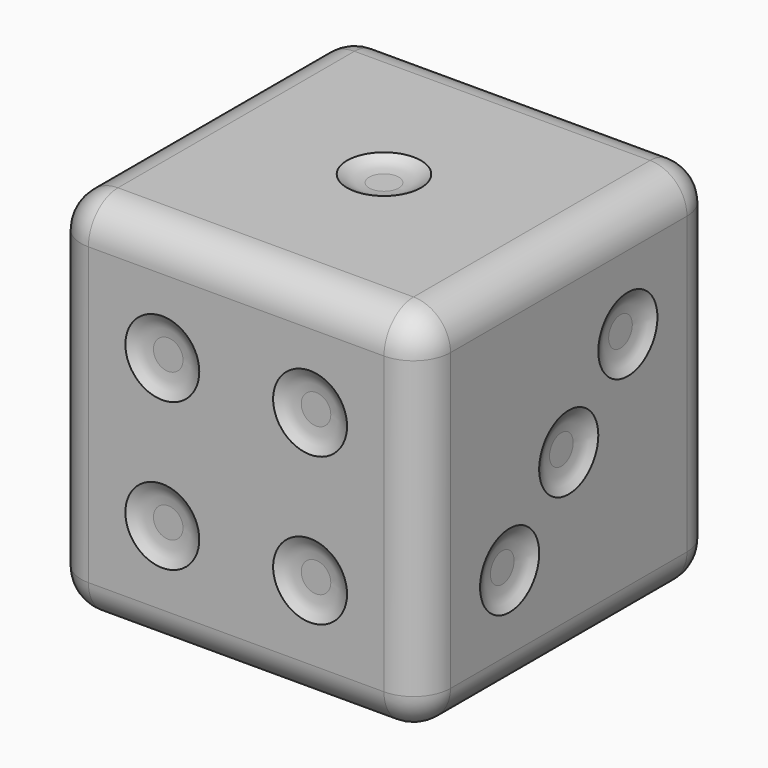
from build123d import *

# Parameters (mm, degrees)
F0_W      = 50
F0_H      = 50
F1_DEPTH  = 50
F2_R      = 5
F3_DEPTH  = 1
F4_R      = 5
F6_R      = 5
F7_DEPTH  = 1
F9_R      = 5
F10_DEPTH = 1
F12_R     = 5
F13_DEPTH = 1
F15_R     = 5
F16_DEPTH = 1
F18_R     = 5
F19_DEPTH = 1
F21_DEPTH = 0.5


# Not quite as in the source:
# - a fillet or chamfer that OpenCascade refuses, or shapes differently, is made with other operations: its cross-section is extruded or revolved along the edge and cut away or added
# - a feature names something its author has since deleted; it is built from what else it names


with BuildPart() as f1:
    # F0 (on Top) → F1 (new body)
    with BuildSketch(Plane.XY):
        with Locations((25, -25)):
            Rectangle(F0_W, F0_H)
    extrude(amount=F1_DEPTH)

    # F2 (on face) → F3 (cut)
    with BuildSketch(Plane.XY.offset(50)):
        with Locations((25, -25)):
            Circle(F2_R)
    extrude(amount=-F3_DEPTH, mode=Mode.SUBTRACT)

    # F4
    f4_edges = [f1.edges().sort_by_distance(p)[0] for p in [
        (0, -50, 25),
        (25, -50, 50),
        (25, 0, 50),
        (0, 0, 25),
        (0, -25, 0),
        (0, -25, 50),
        (25, -50, 0),
        (50, -50, 25),
        (25, 0, 0),
        (50, 0, 25),
        (50, -25, 0),
        (50, -25, 50),
    ]]
    fillet(f4_edges, radius=F4_R)

    # F5: fillet of radius 5 on 1 edges, made by hand

    # F5_s1 → F5_t2 (revolve)
    with BuildSketch(Plane.XZ.offset(25)):
        with BuildLine():
            ThreePointArc((30, 50), (28.5811388301, 49.2565835097), (27, 49))
            Line((27, 49), (30, 49))
            Line((30, 49), (30, 50))
        make_face()
    revolve(axis=Axis((25, -25, 49), (0, 0, 1)))

    # F6 (on face) → F7 (cut)
    with BuildSketch(Plane.XZ.offset(50)):
        with Locations((15, 35)):
            Circle(F6_R)
        with Locations((35, 35)):
            Circle(F6_R)
        with Locations((35, 15)):
            Circle(F6_R)
        with Locations((15, 15)):
            Circle(F6_R)
    extrude(amount=-F7_DEPTH, mode=Mode.SUBTRACT)

    # F8: fillet of radius 5 on 4 edges, made by hand

    # F8_s1 → F8_t2 (revolve)
    with BuildSketch(Plane.XY.offset(35)):
        with BuildLine():
            ThreePointArc((20, -50), (18.5811388301, -49.2565835097), (17, -49))
            Line((17, -49), (20, -49))
            Line((20, -49), (20, -50))
        make_face()
    revolve(axis=Axis((15, -49, 35), (0, -1, 0)))

    # F8_s3 → F8_t4 (revolve)
    with BuildSketch(Plane.XY.offset(35)):
        with BuildLine():
            ThreePointArc((40, -50), (38.5811388301, -49.2565835097), (37, -49))
            Line((37, -49), (40, -49))
            Line((40, -49), (40, -50))
        make_face()
    revolve(axis=Axis((35, -49, 35), (0, -1, 0)))

    # F8_s5 → F8_t6 (revolve)
    with BuildSketch(Plane.XY.offset(15)):
        with BuildLine():
            ThreePointArc((20, -50), (18.5811388301, -49.2565835097), (17, -49))
            Line((17, -49), (20, -49))
            Line((20, -49), (20, -50))
        make_face()
    revolve(axis=Axis((15, -49, 15), (0, -1, 0)))

    # F8_s7 → F8_t8 (revolve)
    with BuildSketch(Plane.XY.offset(15)):
        with BuildLine():
            ThreePointArc((40, -50), (38.5811388301, -49.2565835097), (37, -49))
            Line((37, -49), (40, -49))
            Line((40, -49), (40, -50))
        make_face()
    revolve(axis=Axis((35, -49, 15), (0, -1, 0)))

    # F9 (on face) → F10 (cut)
    with BuildSketch(Plane(origin=(0, 0, 0), x_dir=(-1, 0, 0), z_dir=(0, 1, 0))):
        with Locations((-35, 15)):
            Circle(F9_R)
        with Locations((-15, 35)):
            Circle(F9_R)
    extrude(amount=-F10_DEPTH, mode=Mode.SUBTRACT)

    # F11: fillet of radius 5 on 2 edges, made by hand

    # F11_s1 → F11_t2 (revolve)
    with BuildSketch(Plane.XY.offset(15)):
        with BuildLine():
            ThreePointArc((30, 0), (31.4188611699, -0.7434164903), (33, -1))
            Line((33, -1), (30, -1))
            Line((30, -1), (30, 0))
        make_face()
    revolve(axis=Axis((35, -1, 15), (0, 1, 0)))

    # F11_s3 → F11_t4 (revolve)
    with BuildSketch(Plane.XY.offset(35)):
        with BuildLine():
            ThreePointArc((10, 0), (11.4188611699, -0.7434164903), (13, -1))
            Line((13, -1), (10, -1))
            Line((10, -1), (10, 0))
        make_face()
    revolve(axis=Axis((15, -1, 35), (0, 1, 0)))

    # F12 (on face) → F13 (cut)
    with BuildSketch(Plane.YZ.offset(50)):
        with Locations((-15, 35)):
            Circle(F12_R)
        with Locations((-25, 25)):
            Circle(F12_R)
        with Locations((-35, 15)):
            Circle(F12_R)
    extrude(amount=-F13_DEPTH, mode=Mode.SUBTRACT)

    # F14: fillet of radius 5 on 3 edges, made by hand

    # F14_s1 → F14_t2 (revolve)
    with BuildSketch(Plane.XY.offset(15)):
        with BuildLine():
            ThreePointArc((50, -30), (49.2565835097, -31.4188611699), (49, -33))
            Line((49, -33), (49, -30))
            Line((49, -30), (50, -30))
        make_face()
    revolve(axis=Axis((49, -35, 15), (1, 0, 0)))

    # F14_s3 → F14_t4 (revolve)
    with BuildSketch(Plane.XY.offset(25)):
        with BuildLine():
            ThreePointArc((50, -20), (49.2565835097, -21.4188611699), (49, -23))
            Line((49, -23), (49, -20))
            Line((49, -20), (50, -20))
        make_face()
    revolve(axis=Axis((49, -25, 25), (1, 0, 0)))

    # F14_s5 → F14_t6 (revolve)
    with BuildSketch(Plane.XY.offset(35)):
        with BuildLine():
            ThreePointArc((50, -10), (49.2565835097, -11.4188611699), (49, -13))
            Line((49, -13), (49, -10))
            Line((49, -10), (50, -10))
        make_face()
    revolve(axis=Axis((49, -15, 35), (1, 0, 0)))

    # F15 (on face) → F16 (cut)
    with BuildSketch(Plane(origin=(0, 0, 0), x_dir=(0, -1, 0), z_dir=(-1, 0, 0))):
        with Locations((15, 35)):
            Circle(F15_R)
        with Locations((25, 25)):
            Circle(F15_R)
        with Locations((15, 15)):
            Circle(F15_R)
        with Locations((35, 15)):
            Circle(F15_R)
        with Locations((35, 35)):
            Circle(F15_R)
    extrude(amount=-F16_DEPTH, mode=Mode.SUBTRACT)

    # F17: fillet of radius 5 on 5 edges, made by hand

    # F17_s1 → F17_t2 (revolve)
    with BuildSketch(Plane.XY.offset(35)):
        with BuildLine():
            ThreePointArc((0, -20), (0.7434164903, -18.5811388301), (1, -17))
            Line((1, -17), (1, -20))
            Line((1, -20), (0, -20))
        make_face()
    revolve(axis=Axis((1, -15, 35), (-1, 0, 0)))

    # F17_s3 → F17_t4 (revolve)
    with BuildSketch(Plane.XY.offset(25)):
        with BuildLine():
            ThreePointArc((0, -30), (0.7434164903, -28.5811388301), (1, -27))
            Line((1, -27), (1, -30))
            Line((1, -30), (0, -30))
        make_face()
    revolve(axis=Axis((1, -25, 25), (-1, 0, 0)))

    # F17_s5 → F17_t6 (revolve)
    with BuildSketch(Plane.XY.offset(15)):
        with BuildLine():
            ThreePointArc((0, -40), (0.7434164903, -38.5811388301), (1, -37))
            Line((1, -37), (1, -40))
            Line((1, -40), (0, -40))
        make_face()
    revolve(axis=Axis((1, -35, 15), (-1, 0, 0)))

    # F17_s7 → F17_t8 (revolve)
    with BuildSketch(Plane.XY.offset(35)):
        with BuildLine():
            ThreePointArc((0, -40), (0.7434164903, -38.5811388301), (1, -37))
            Line((1, -37), (1, -40))
            Line((1, -40), (0, -40))
        make_face()
    revolve(axis=Axis((1, -35, 35), (-1, 0, 0)))

    # F17_s9 → F17_t10 (revolve)
    with BuildSketch(Plane.XY.offset(15)):
        with BuildLine():
            ThreePointArc((0, -20), (0.7434164903, -18.5811388301), (1, -17))
            Line((1, -17), (1, -20))
            Line((1, -20), (0, -20))
        make_face()
    revolve(axis=Axis((1, -15, 15), (-1, 0, 0)))

    # F18 (on face) → F19 (cut)
    with BuildSketch(Plane(origin=(0, 0, 0), x_dir=(1, 0, 0), z_dir=(0, 0, -1))):
        with Locations((15, 37)):
            Circle(F18_R)
        with Locations((15, 25)):
            Circle(F18_R)
        with Locations((15, 13)):
            Circle(F18_R)
        with Locations((35, 37)):
            Circle(F18_R)
        with Locations((35, 13)):
            Circle(F18_R)
        with Locations((35, 25)):
            Circle(F18_R)
    extrude(amount=-F19_DEPTH, mode=Mode.SUBTRACT)

    # F20: fillet of radius 5 on 6 edges, made by hand

    # F20_s1 → F20_t2 (revolve)
    with BuildSketch(Plane.XZ.offset(25)):
        with BuildLine():
            ThreePointArc((40, 0), (38.5811388301, 0.7434164903), (37, 1))
            Line((37, 1), (40, 1))
            Line((40, 1), (40, 0))
        make_face()
    revolve(axis=Axis((35, -25, 1), (0, 0, -1)))

    # F20_s3 → F20_t4 (revolve)
    with BuildSketch(Plane.XZ.offset(25)):
        with BuildLine():
            ThreePointArc((20, 0), (18.5811388301, 0.7434164903), (17, 1))
            Line((17, 1), (20, 1))
            Line((20, 1), (20, 0))
        make_face()
    revolve(axis=Axis((15, -25, 1), (0, 0, -1)))

    # F20_s5 → F20_t6 (revolve)
    with BuildSketch(Plane.XZ.offset(37)):
        with BuildLine():
            ThreePointArc((20, 0), (18.5811388301, 0.7434164903), (17, 1))
            Line((17, 1), (20, 1))
            Line((20, 1), (20, 0))
        make_face()
    revolve(axis=Axis((15, -37, 1), (0, 0, -1)))

    # F20_s7 → F20_t8 (revolve)
    with BuildSketch(Plane.XZ.offset(13)):
        with BuildLine():
            ThreePointArc((20, 0), (18.5811388301, 0.7434164903), (17, 1))
            Line((17, 1), (20, 1))
            Line((20, 1), (20, 0))
        make_face()
    revolve(axis=Axis((15, -13, 1), (0, 0, -1)))

    # F20_s9 → F20_t10 (revolve)
    with BuildSketch(Plane.XZ.offset(13)):
        with BuildLine():
            ThreePointArc((40, 0), (38.5811388301, 0.7434164903), (37, 1))
            Line((37, 1), (40, 1))
            Line((40, 1), (40, 0))
        make_face()
    revolve(axis=Axis((35, -13, 1), (0, 0, -1)))

    # F20_s11 → F20_t12 (revolve)
    with BuildSketch(Plane.XZ.offset(37)):
        with BuildLine():
            ThreePointArc((40, 0), (38.5811388301, 0.7434164903), (37, 1))
            Line((37, 1), (40, 1))
            Line((40, 1), (40, 0))
        make_face()
    revolve(axis=Axis((35, -37, 1), (0, 0, -1)))

    # F21 (add): a face of the model
    f21_faces = [f1.faces().sort_by_distance(p)[0] for p in [
        (25, -25, 0),
    ]]
    extrude(f21_faces, amount=-F21_DEPTH)


solid = f1.part
